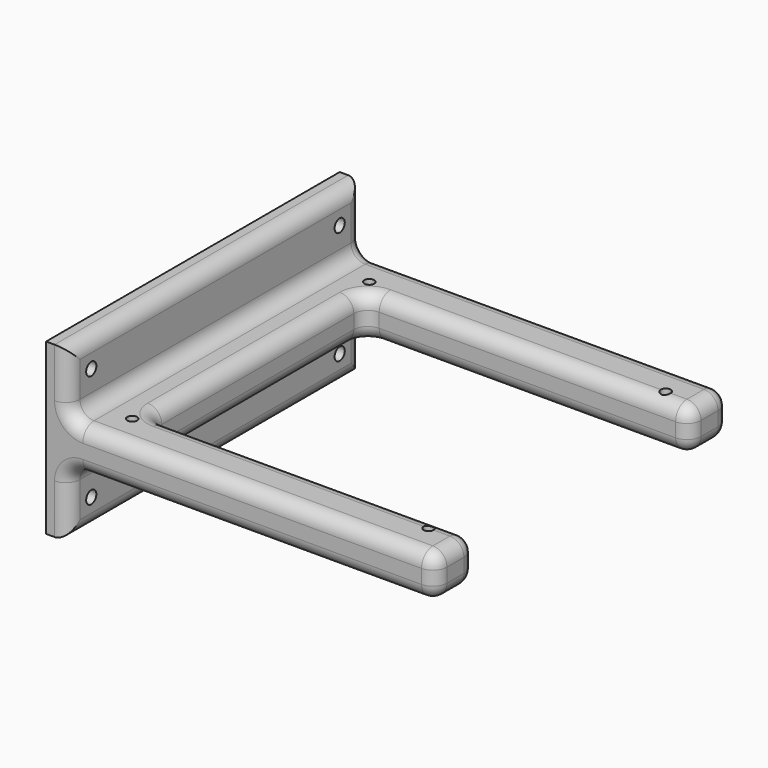
from build123d import *

# Parameters (mm, degrees)
F0_R         = 1.75
F1_DEPTH     = 15
F2_W         = 130
F2_H         = 22.5
F2_R         = 2.25
F3_DEPTH     = 8
F4_F1_R      = 5
F4_F2_R      = 5
F4_T3_DEPTH  = 105
F4_T5_DEPTH  = 85
F4_S9_W      = 5.1
F4_S9_H      = 5.1
F4_T10_DEPTH = 5.1
F4_S15_W     = 5.1
F4_S15_H     = 5.1
F4_T16_DEPTH = 5.1
F4_S21_W     = 5.1
F4_S21_H     = 5.1
F4_T22_DEPTH = 5.1
F4_S27_W     = 5.1
F4_S27_H     = 5.1
F4_T28_DEPTH = 5.1
F4_T32_ANGLE = 90
F4_T34_ANGLE = 90
F4_T36_ANGLE = 90
F4_T38_ANGLE = 90


# Not quite as in the source:
# - a fillet or chamfer that OpenCascade refuses, or shapes differently, is made with other operations: its cross-section is extruded or revolved along the edge and cut away or added


with BuildPart() as f1:
    # F0 (on Top) → F1 (new body)
    with BuildSketch(Plane.XY):
        Polygon((0, 130), (0, 0), (130, 0), (130, 17.5), (15, 17.5), (15, 112.5), (130, 112.5), (130, 130), align=None)
        with Locations((12.5, 12.5)):
            Circle(F0_R, mode=Mode.SUBTRACT)
        with Locations((117.5, 12.5)):
            Circle(F0_R, mode=Mode.SUBTRACT)
        with Locations((12.5, 117.5)):
            Circle(F0_R, mode=Mode.SUBTRACT)
        with Locations((117.5, 117.5)):
            Circle(F0_R, mode=Mode.SUBTRACT)
    extrude(amount=F1_DEPTH)

    # F2 (on face) → F3 (join)
    with BuildSketch(Plane(origin=(0, 0, 0), x_dir=(0, -1, 0), z_dir=(-1, 0, 0))):
        with Locations((-65, -11.25)):
            Rectangle(F2_W, F2_H)
        with Locations((-120, -12.5)):
            Circle(F2_R, mode=Mode.SUBTRACT)
        with Locations((-10, -12.5)):
            Circle(F2_R, mode=Mode.SUBTRACT)
        Polygon((0, 15), (-130, 15), (-130, 7.5), (-130, 0), (0, 0), (0, 7.5), align=None)
        with Locations((-65, 26.25)):
            Rectangle(F2_W, F2_H)
        with Locations((-120, 27.5)):
            Circle(F2_R, mode=Mode.SUBTRACT)
        with Locations((-10, 27.5)):
            Circle(F2_R, mode=Mode.SUBTRACT)
    extrude(amount=F3_DEPTH)

    # F4: fillet of radius 5 on 24 edges, made by hand

    # F4_f1
    f4_f1_edges = [f1.edges().sort_by_distance(p)[0] for p in [
        (0, 65, 15),
        (0, 65, 0),
        (15, 112.5, 7.5),
        (15, 17.5, 7.5),
    ]]
    fillet(f4_f1_edges, radius=F4_F1_R)

    # F4_f2
    f4_f2_edges = [f1.edges().sort_by_distance(p)[0] for p in [
        (130, 17.5, 7.5),
        (130, 0, 7.5),
        (130, 130, 7.5),
        (130, 112.5, 7.5),
        (67.5, 0, 15),
        (67.5, 130, 15),
        (0, 65, 37.5),
        (67.5, 0, 0),
        (0, 65, -22.5),
        (67.5, 130, 0),
        (130, 8.75, 15),
        (130, 121.25, 15),
        (130, 8.75, 0),
        (130, 121.25, 0),
        (1.4644660941, 130, -1.4644660941),
        (1.4644660941, 0, -1.4644660941),
        (1.4644660941, 130, 16.4644660941),
        (1.4644660941, 0, 16.4644660941),
    ]]
    fillet(f4_f2_edges, radius=F4_F2_R)

    # F4_s4 → F4_t3 (cut)
    with BuildSketch(Plane.YZ.offset(20)):
        with BuildLine():
            ThreePointArc((117.5, 15), (113.9644660941, 13.5355339059), (112.5, 10))
            Line((112.5, 10), (112.4, 10))
            Line((112.4, 10), (112.4, 15.1))
            Line((112.4, 15.1), (117.5, 15.1))
            Line((117.5, 15.1), (117.5, 15))
        make_face()
        with BuildLine():
            ThreePointArc((117.5, 0), (113.9644660941, 1.4644660941), (112.5, 5))
            Line((112.5, 5), (112.4, 5))
            Line((112.4, 5), (112.4, -0.1))
            Line((112.4, -0.1), (117.5, -0.1))
            Line((117.5, -0.1), (117.5, 0))
        make_face()
        with BuildLine():
            ThreePointArc((12.5, 0), (16.0355339059, 1.4644660941), (17.5, 5))
            Line((17.5, 5), (17.6, 5))
            Line((17.6, 5), (17.6, -0.1))
            Line((17.6, -0.1), (12.5, -0.1))
            Line((12.5, -0.1), (12.5, 0))
        make_face()
        with BuildLine():
            ThreePointArc((12.5, 15), (16.0355339059, 13.5355339059), (17.5, 10))
            Line((17.5, 10), (17.6, 10))
            Line((17.6, 10), (17.6, 15.1))
            Line((17.6, 15.1), (12.5, 15.1))
            Line((12.5, 15.1), (12.5, 15))
        make_face()
    extrude(amount=F4_T3_DEPTH, mode=Mode.SUBTRACT)

    # F4_s6 → F4_t5 (cut)
    with BuildSketch(Plane.XZ.offset(-107.5)):
        with BuildLine():
            ThreePointArc((10, 0), (13.5355339059, 1.4644660941), (15, 5))
            Line((15, 5), (15.1, 5))
            Line((15.1, 5), (15.1, -0.1))
            Line((15.1, -0.1), (10, -0.1))
            Line((10, -0.1), (10, 0))
        make_face()
        with BuildLine():
            ThreePointArc((10, 15), (13.5355339059, 13.5355339059), (15, 10))
            Line((15, 10), (15.1, 10))
            Line((15.1, 10), (15.1, 15.1))
            Line((15.1, 15.1), (10, 15.1))
            Line((10, 15.1), (10, 15))
        make_face()
    extrude(amount=F4_T5_DEPTH, mode=Mode.SUBTRACT)


with BuildPart() as f4_tool8:
    # F4_s9 → F4_t10 (new body)
    with BuildSketch(Plane.XY.offset(10)):
        with Locations((127.55, 15.05)):
            Rectangle(F4_S9_W, F4_S9_H)
    extrude(amount=F4_T10_DEPTH)

    # F4_s11 → F4_t12 (revolve, cut)
    with BuildSketch(Plane(origin=(125, 12.5, 10), x_dir=(-0.7071067812, -0.7071067812, 0), z_dir=(-0.7071067812, 0.7071067812, 0))):
        with BuildLine():
            ThreePointArc((0, -5), (5, 0), (0, 5))
            Line((0, 5), (0, -5))
        make_face()
    revolve(axis=Axis((125, 12.5, 10), (0, 0, 1)), mode=Mode.SUBTRACT)


with BuildPart() as f1_1:
    add(f1.part)

    # F4_t7: cut F4_tool8
    add(f4_tool8.part, mode=Mode.SUBTRACT)


with BuildPart() as f4_tool14:
    # F4_s15 → F4_t16 (new body)
    with BuildSketch(Plane.XY.offset(5)):
        with Locations((127.55, 15.05)):
            Rectangle(F4_S15_W, F4_S15_H)
    extrude(amount=-F4_T16_DEPTH)

    # F4_s17 → F4_t18 (revolve, cut)
    with BuildSketch(Plane(origin=(125, 12.5, 5), x_dir=(-0.7071067812, -0.7071067812, 0), z_dir=(0.7071067812, -0.7071067812, 0))):
        with BuildLine():
            ThreePointArc((0, -5), (5, 0), (0, 5))
            Line((0, 5), (0, -5))
        make_face()
    revolve(axis=Axis((125, 12.5, 5), (0, 0, -1)), mode=Mode.SUBTRACT)


with BuildPart() as f1_2:
    add(f1_1.part)

    # F4_t13: cut F4_tool14
    add(f4_tool14.part, mode=Mode.SUBTRACT)


with BuildPart() as f4_tool20:
    # F4_s21 → F4_t22 (new body)
    with BuildSketch(Plane.XY.offset(5)):
        with Locations((127.55, 114.95)):
            Rectangle(F4_S21_W, F4_S21_H)
    extrude(amount=-F4_T22_DEPTH)

    # F4_s23 → F4_t24 (revolve, cut)
    with BuildSketch(Plane(origin=(125, 117.5, 5), x_dir=(-0.7071067812, 0.7071067812, 0), z_dir=(-0.7071067812, -0.7071067812, 0))):
        with BuildLine():
            ThreePointArc((0, -5), (5, 0), (0, 5))
            Line((0, 5), (0, -5))
        make_face()
    revolve(axis=Axis((125, 117.5, 5), (0, 0, -1)), mode=Mode.SUBTRACT)


with BuildPart() as f1_3:
    add(f1_2.part)

    # F4_t19: cut F4_tool20
    add(f4_tool20.part, mode=Mode.SUBTRACT)


with BuildPart() as f4_tool26:
    # F4_s27 → F4_t28 (new body)
    with BuildSketch(Plane.XY.offset(10)):
        with Locations((127.55, 114.95)):
            Rectangle(F4_S27_W, F4_S27_H)
    extrude(amount=F4_T28_DEPTH)

    # F4_s29 → F4_t30 (revolve, cut)
    with BuildSketch(Plane(origin=(125, 117.5, 10), x_dir=(-0.7071067812, 0.7071067812, 0), z_dir=(0.7071067812, 0.7071067812, 0))):
        with BuildLine():
            ThreePointArc((0, -5), (5, 0), (0, 5))
            Line((0, 5), (0, -5))
        make_face()
    revolve(axis=Axis((125, 117.5, 10), (0, 0, 1)), mode=Mode.SUBTRACT)


with BuildPart() as f1_4:
    add(f1_3.part)

    # F4_t25: cut F4_tool26
    add(f4_tool26.part, mode=Mode.SUBTRACT)

    # F4_s31 → F4_t32 (revolve, cut)
    with BuildSketch(Plane.YZ.offset(20)):
        with BuildLine():
            ThreePointArc((12.5, 15), (16.0355339059, 13.5355339059), (17.5, 10))
            Line((17.5, 10), (17.6, 10))
            Line((17.6, 10), (17.6, 15.1))
            Line((17.6, 15.1), (12.5, 15.1))
            Line((12.5, 15.1), (12.5, 15))
        make_face()
    revolve(axis=Axis((20, 22.5, 15), (0, 0, -1)), revolution_arc=F4_T32_ANGLE, mode=Mode.SUBTRACT)

    # F4_s33 → F4_t34 (revolve, cut)
    with BuildSketch(Plane.XZ.offset(-107.5)):
        with BuildLine():
            ThreePointArc((10, 15), (13.5355339059, 13.5355339059), (15, 10))
            Line((15, 10), (15.1, 10))
            Line((15.1, 10), (15.1, 15.1))
            Line((15.1, 15.1), (10, 15.1))
            Line((10, 15.1), (10, 15))
        make_face()
    revolve(axis=Axis((20, 107.5, 15), (0, 0, -1)), revolution_arc=F4_T34_ANGLE, mode=Mode.SUBTRACT)

    # F4_s35 → F4_t36 (revolve, cut)
    with BuildSketch(Plane.YZ.offset(20)):
        with BuildLine():
            ThreePointArc((12.5, 0), (16.0355339059, 1.4644660941), (17.5, 5))
            Line((17.5, 5), (17.6, 5))
            Line((17.6, 5), (17.6, -0.1))
            Line((17.6, -0.1), (12.5, -0.1))
            Line((12.5, -0.1), (12.5, 0))
        make_face()
    revolve(axis=Axis((20, 22.5, 0), (0, 0, -1)), revolution_arc=F4_T36_ANGLE, mode=Mode.SUBTRACT)

    # F4_s37 → F4_t38 (revolve, cut)
    with BuildSketch(Plane.XZ.offset(-107.5)):
        with BuildLine():
            ThreePointArc((10, 0), (13.5355339059, 1.4644660941), (15, 5))
            Line((15, 5), (15.1, 5))
            Line((15.1, 5), (15.1, -0.1))
            Line((15.1, -0.1), (10, -0.1))
            Line((10, -0.1), (10, 0))
        make_face()
    revolve(axis=Axis((20, 107.5, 0), (0, 0, -1)), revolution_arc=F4_T38_ANGLE, mode=Mode.SUBTRACT)


solid = f1_4.part
